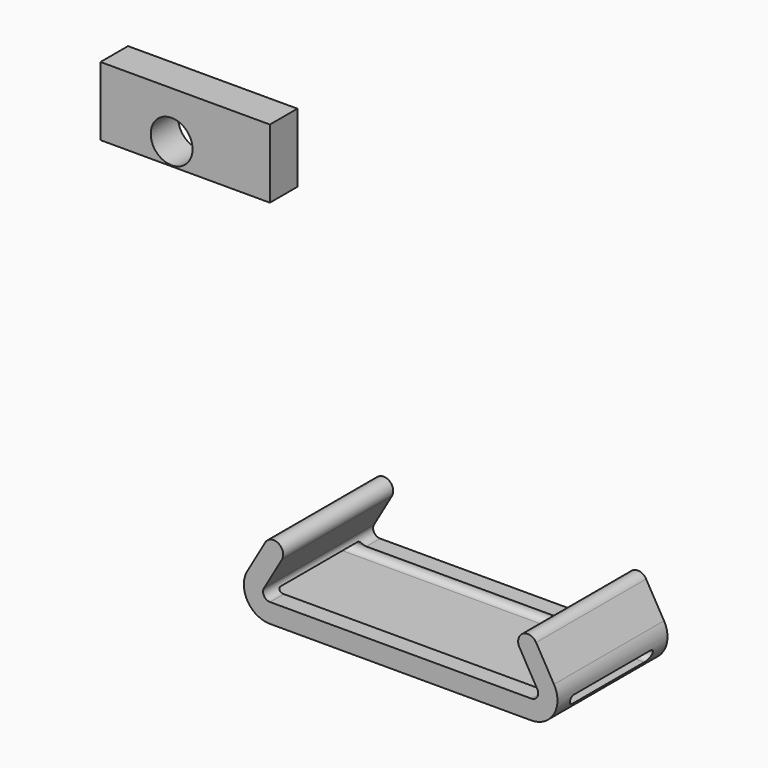
from build123d import *

# Parameters (mm, degrees)
F1_DEPTH = 20
F2_W     = 15
F2_H     = 1.5
F3_DEPTH = 25
F4_R     = 0.99999
F5_R     = 0.5
F6_W     = 24.6281530708
F6_H     = 10.0072175264
F7_DEPTH = 5
F8_R     = 3.0398378779
F9_DEPTH = 25


# Not quite as in the source:
# - a fillet or chamfer is up to 0.001 mm smaller than in the source, because OpenCascade refuses the exact size


with BuildPart() as f1:
    # F0 (on Front) → F1 (new body)
    with BuildSketch(Plane.XZ):
        with BuildLine():
            Line((19, 0), (0, 0))
            Line((0, 0), (-19, 0))
            ThreePointArc((-19, 0), (-19.8660254038, 0.5), (-19.8660254038, 1.5))
            Line((-19.8660254038, 1.5), (-17.2679491924, 6))
            ThreePointArc((-17.2679491924, 6), (-17.7803847577, 7.9124355653), (-19.692820323, 7.4))
            Line((-19.692820323, 7.4), (-22.2908965344, 2.9))
            ThreePointArc((-22.2908965344, 2.9), (-22.2908965344, -0.9), (-19, -2.8))
            Line((-19, -2.8), (0, -2.8))
            Line((0, -2.8), (19, -2.8))
            ThreePointArc((19, -2.8), (22.2908965344, -0.9), (22.2908965344, 2.9))
            Line((22.2908965344, 2.9), (19.692820323, 7.4))
            ThreePointArc((19.692820323, 7.4), (17.7803847577, 7.9124355653), (17.2679491924, 6))
            Line((17.2679491924, 6), (19.8660254038, 1.5))
            ThreePointArc((19.8660254038, 1.5), (19.8660254038, 0.5), (19, 0))
        make_face()
    extrude(amount=F1_DEPTH)

    # F2 (on Right) → F3 (cut, symmetric)
    with BuildSketch(Plane.YZ):
        with Locations((-10, -0.25)):
            Rectangle(F2_W, F2_H)
    extrude(amount=F3_DEPTH, both=True, mode=Mode.SUBTRACT)

    # F4 (radius 1 in the source; OpenCascade refuses exactly that, so slightly less here)
    f4_edges = [f1.edges().sort_by_distance(p)[0] for p in [
        (0, -17.5, -1),
        (0, -2.5, -1),
    ]]
    fillet(f4_edges, radius=F4_R)

    # F5
    f5_edges = [f1.edges().sort_by_distance(p)[0] for p in [
        (21.316494, -17.5, 0.5),
        (21.316494, -2.5, 0.5),
        (-21.316494, -17.5, 0.5),
        (-21.316494, -2.5, 0.5),
    ]]
    fillet(f5_edges, radius=F5_R)


with BuildPart() as f7:
    # F6 (on Front) → F7 (new body)
    with BuildSketch(Plane.XZ):
        with Locations((-43.3283532038, 46.11190781)):
            Rectangle(F6_W, F6_H)
    extrude(amount=F7_DEPTH)

    # F8 (on face) → F9 (cut)
    with BuildSketch(Plane.XZ.offset(5)):
        with Locations((-45.3025065362, 44.2891865969)):
            Circle(F8_R)
    extrude(amount=-F9_DEPTH, mode=Mode.SUBTRACT)


solid = Compound([f1.part, f7.part])
